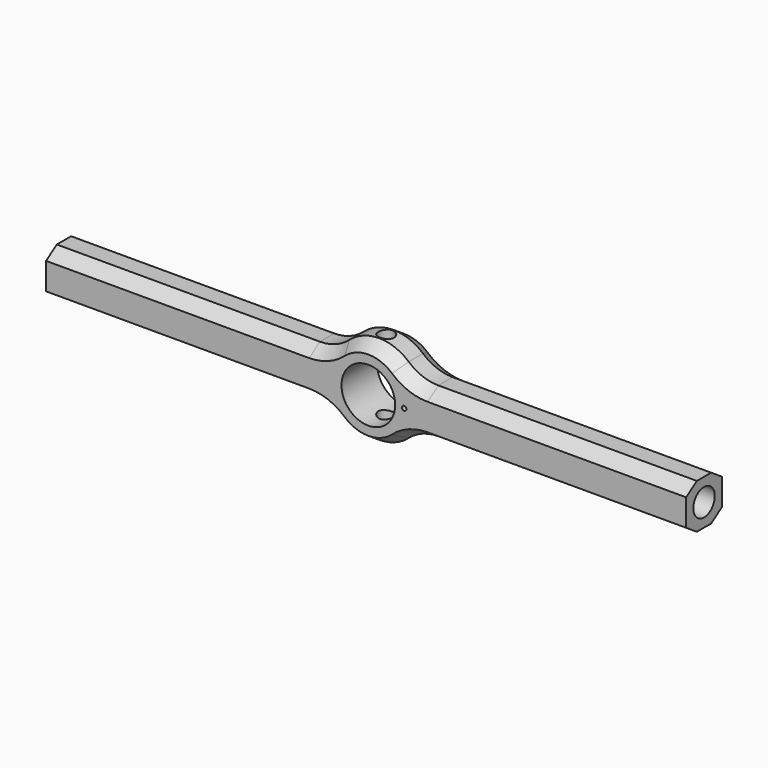
from build123d import *

# Parameters (mm, degrees)
F0_R          = 6
F0_R_2        = 0.5
F1_DEPTH      = 10
F2_R          = 3
F3_DEPTH      = 40
F4_R          = 1.75
F5_DEPTH      = 10.001
F5_DEPTH_BACK = 10.001
F6_R          = 10
F7_SIZE2      = 3
F7_SIZE       = 2
F7_2_SIZE2    = 3
F7_2_SIZE     = 2


# Not quite as in the source:
# - a pattern or mirror of a feature is missing from the dataset's text; its kind, count and spacing are read off the source's solid


with BuildPart() as f1:
    # F0 (on Front) → F1 (new body)
    with BuildSketch(Plane.XZ):
        with BuildLine():
            Line((71, 5), (8.6602540378, 5))
            ThreePointArc((8.6602540378, 5), (0, 10), (-8.6602540378, 5))
            Line((-8.6602540378, 5), (-72, 5))
            Line((-72, 5), (-72, -5))
            Line((-72, -5), (-8.6602540378, -5))
            ThreePointArc((-8.6602540378, -5), (0, -10), (8.6602540378, -5))
            Line((8.6602540378, -5), (71, -5))
            Line((71, -5), (71, 5))
        make_face()
        Circle(F0_R, mode=Mode.SUBTRACT)
        with Locations((8, 0)):
            Circle(F0_R_2, mode=Mode.SUBTRACT)
    extrude(amount=F1_DEPTH)

    # F2 (on face) → F3 (cut)
    with BuildSketch(Plane(origin=(-72, 0, 0), x_dir=(0, -1, 0), z_dir=(-1, 0, 0))):
        with Locations((5, 0)):
            Circle(F2_R)
    f3 = extrude(amount=-F3_DEPTH, mode=Mode.SUBTRACT)

    # F3_copies: F3 across plane
    add(f3.mirror(Plane(origin=(0, 0, 0), x_dir=(0, 0, 1), z_dir=(1, 0, 0))), mode=Mode.SUBTRACT)

    # F4 (on Top) → F5 (cut, two sides)
    with BuildSketch(Plane.XY) as f5_sk:
        with Locations((0, -5)):
            Circle(F4_R)
    extrude(amount=-F5_DEPTH, mode=Mode.SUBTRACT)
    extrude(f5_sk.sketch, amount=F5_DEPTH_BACK, mode=Mode.SUBTRACT)

    # F6
    f6_edges = [f1.edges().sort_by_distance(p)[0] for p in [
        (-8.660254, -5, 5),
        (8.660254, -5, 5),
        (8.660254, -5, -5),
        (-8.660254, -5, -5),
    ]]
    fillet(f6_edges, radius=F6_R)

    # F7
    f7_edges = [f1.edges().sort_by_distance(p)[0] for p in [
        (-42.614378, -10, 5),
        (-42.614378, -10, -5),
    ]]
    f7_side = f1.faces().sort_by_distance((42.114378, -10, -3.556082))[0]
    chamfer(f7_edges, length=F7_SIZE, length2=F7_SIZE2, reference=f7_side)

    # F7#2
    f7_2_edges = [f1.edges().sort_by_distance(p)[0] for p in [
        (-42.614378, 0, 5),
        (-42.614378, 0, -5),
    ]]
    f7_2_side = f1.faces().sort_by_distance((42.114378, 0, -3.556082))[0]
    chamfer(f7_2_edges, length=F7_2_SIZE, length2=F7_2_SIZE2, reference=f7_2_side)


solid = f1.part
